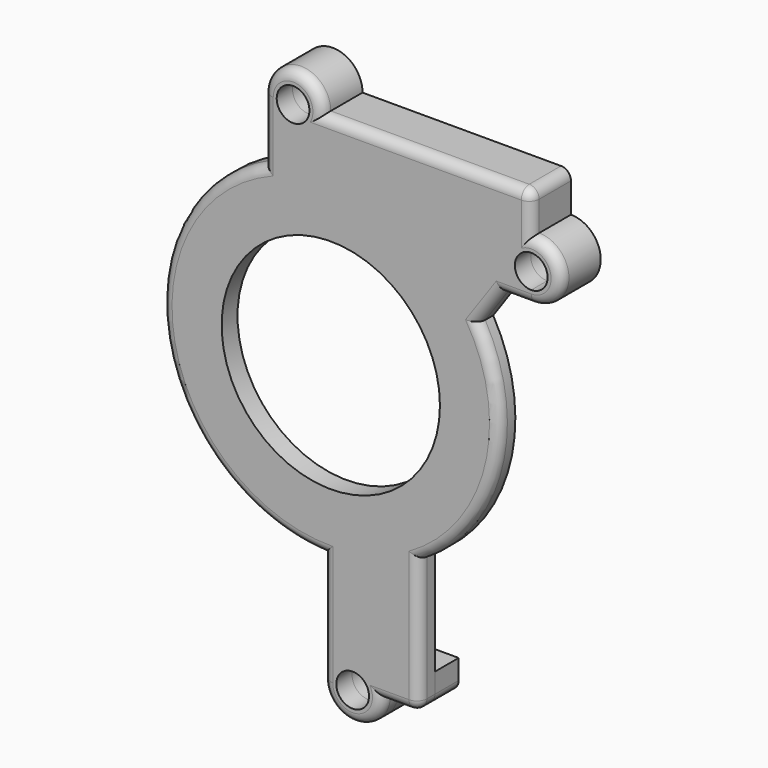
from build123d import *

# Parameters (mm, degrees)
F0_R     = 11
F1_DEPTH = 2
F2_DEPTH = 3
F3_R     = 1


with BuildPart() as f1:
    # F0 (on Front) → F1 (new body)
    with BuildSketch(Plane.XZ):
        with BuildLine():
            Line((38, 47), (38, 44))
            Line((38, 44), (62, 44))
            Line((62, 44), (62, 37))
            Line((62, 37), (65, 37))
            Line((65, 37), (65, 38.35))
            ThreePointArc((65, 38.35), (63.35, 40), (65, 41.65))
            Line((65, 41.65), (65, 43))
            Line((65, 43), (65, 47))
            Line((65, 47), (44, 47))
            Line((44, 47), (42.65, 47))
            ThreePointArc((42.65, 47), (41, 45.35), (39.35, 47))
            Line((39.35, 47), (38, 47))
        make_face()
        with BuildLine():
            ThreePointArc((44, 47), (41, 50), (38, 47))
            Line((38, 47), (39.35, 47))
            ThreePointArc((39.35, 47), (41, 48.65), (42.65, 47))
            Line((42.65, 47), (44, 47))
        make_face()
        with BuildLine():
            Line((62, 44), (38, 44))
            Line((38, 44), (38, 40.6807573628))
            ThreePointArc((38, 40.6807573628), (28.0814559879, 22.0193692019), (44, 8.1188339623))
            Line((44, 8.1188339623), (44, 0))
            Line((44, 0), (53.6880180275, 0))
            Line((53.6880180275, 0), (53.6880180275, 10.6085150677))
            ThreePointArc((53.6880180275, 10.6085150677), (61.2664808606, 20.8744813256), (59.5676963486, 33.5211130236))
            Line((59.5676963486, 33.5211130236), (62, 37))
            Line((62, 37), (62, 44))
        make_face()
        with Locations((44.8, 25.1)):
            Circle(F0_R, mode=Mode.SUBTRACT)
        with BuildLine():
            Line((53.6880180275, 0), (44, 0))
            Line((44, 0), (44, -3))
            Line((44, -3), (45.35, -3))
            ThreePointArc((45.35, -3), (47, -1.35), (48.65, -3))
            Line((48.65, -3), (50, -3))
            Line((50, -3), (53.6880180275, -3))
            Line((53.6880180275, -3), (53.6880180275, 0))
        make_face()
        with BuildLine():
            Line((45.35, -3), (44, -3))
            ThreePointArc((44, -3), (47, -6), (50, -3))
            Line((50, -3), (48.65, -3))
            ThreePointArc((48.65, -3), (47, -4.65), (45.35, -3))
        make_face()
        with BuildLine():
            Line((65, 38.35), (65, 37))
            ThreePointArc((65, 37), (68, 40), (65, 43))
            Line((65, 43), (65, 41.65))
            ThreePointArc((65, 41.65), (66.166726189, 41.166726189), (66.65, 40))
            ThreePointArc((66.65, 40), (66.166726189, 38.833273811), (65, 38.35))
        make_face()
    extrude(amount=F1_DEPTH)

    # F0 (on Front) → F2 (join)
    with BuildSketch(Plane.XZ):
        with BuildLine():
            ThreePointArc((44, 47), (41, 50), (38, 47))
            Line((38, 47), (39.35, 47))
            ThreePointArc((39.35, 47), (41, 48.65), (42.65, 47))
            Line((42.65, 47), (44, 47))
        make_face()
        with BuildLine():
            Line((38, 47), (38, 44))
            Line((38, 44), (62, 44))
            Line((62, 44), (62, 37))
            Line((62, 37), (65, 37))
            Line((65, 37), (65, 38.35))
            ThreePointArc((65, 38.35), (63.35, 40), (65, 41.65))
            Line((65, 41.65), (65, 43))
            Line((65, 43), (65, 47))
            Line((65, 47), (44, 47))
            Line((44, 47), (42.65, 47))
            ThreePointArc((42.65, 47), (41, 45.35), (39.35, 47))
            Line((39.35, 47), (38, 47))
        make_face()
        with BuildLine():
            Line((65, 38.35), (65, 37))
            ThreePointArc((65, 37), (68, 40), (65, 43))
            Line((65, 43), (65, 41.65))
            ThreePointArc((65, 41.65), (66.166726189, 41.166726189), (66.65, 40))
            ThreePointArc((66.65, 40), (66.166726189, 38.833273811), (65, 38.35))
        make_face()
        with BuildLine():
            Line((45.35, -3), (44, -3))
            ThreePointArc((44, -3), (47, -6), (50, -3))
            Line((50, -3), (48.65, -3))
            ThreePointArc((48.65, -3), (47, -4.65), (45.35, -3))
        make_face()
        with BuildLine():
            Line((53.6880180275, 0), (44, 0))
            Line((44, 0), (44, -3))
            Line((44, -3), (45.35, -3))
            ThreePointArc((45.35, -3), (47, -1.35), (48.65, -3))
            Line((48.65, -3), (50, -3))
            Line((50, -3), (53.6880180275, -3))
            Line((53.6880180275, -3), (53.6880180275, 0))
        make_face()
    extrude(amount=-F2_DEPTH)

    # F3
    f3_edges = [f1.edges().sort_by_distance(p)[0] for p in [
        (38, -2, 43.840379),
        (41, -2, 50),
        (54.5, -2, 47),
        (65, -2, 45),
        (68, -2, 40),
        (63.5, -2, 37),
        (60.783848, -2, 35.260557),
        (61.266481, -2, 20.874481),
        (44, -2, 2.559417),
        (47, -2, -6),
        (51.844009, -2, -3),
        (53.688018, -2, 3.804258),
        (65, 0.5, 47),
        (53.688018, 0.5, -3),
        (28.081456, -2, 22.019369),
    ]]
    fillet(f3_edges, radius=F3_R)


solid = f1.part
